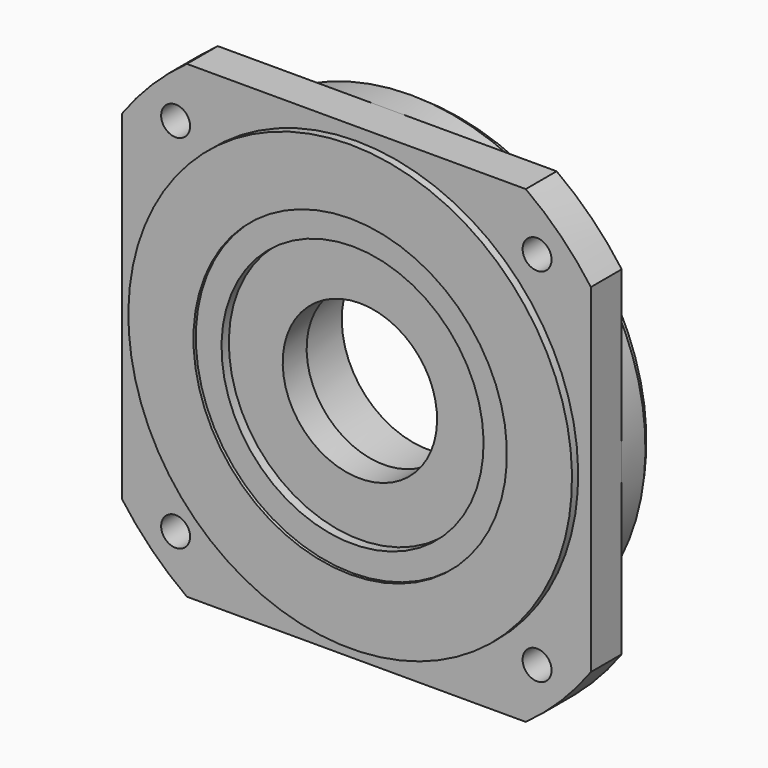
from build123d import *

# Parameters (mm, degrees)
F2_R            = 7.5
F3_DEPTH        = 25.4
F3_COPIES_COUNT = 4
F4_R            = 12.7


# Not quite as in the source:
# - a pattern or mirror of a feature is missing from the dataset's text; its kind, count and spacing are read off the source's solid


with BuildPart() as f1:
    # F0 (on Right) → F1 (revolve)
    with BuildSketch(Plane.YZ):
        Polygon((23.9776, 150), (3.9878, 150), (3.9878, 114.9985), (0, 114.9985), (0, 81.2514126301), (1.524, 81.2514126301), (1.524, 67.9329782724), (6.2865, 67.9329782724), (6.2865, 40.0177), (21.7932, 40.0177), (21.7932, 45.0088), (50.8, 45.0088), (50.8, 51.3588), (12.7, 54.6921180803), (12.7, 113.4999), (44.1452, 113.4999), (44.1452, 118.2624), (39.37, 118.2624), (39.37, 121.5898), (23.9776, 121.5898), align=None)
    revolve(axis=Axis((0, 63.4710703942, 0), (0, 1, 0)))

    # F2 (on face) → F3 (cut)
    with BuildSketch(Plane.XZ.offset(-3.9878)):
        with Locations((-93.6910121111, 93.6910121111)):
            Circle(F2_R)
        with BuildLine():
            Line((-111.0230386257, 169.054677367), (-111.0230386257, 121.5898))
            Line((-111.0230386257, 121.5898), (-87.8403127041, 121.5898))
            ThreePointArc((-87.8403127041, 121.5898), (0, 150), (87.8403127041, 121.5898))
            Line((87.8403127041, 121.5898), (147.7070748806, 121.5898))
            Line((147.7070748806, 121.5898), (147.7070748806, 169.054677367))
            Line((147.7070748806, 169.054677367), (-111.0230386257, 169.054677367))
        make_face()
        with BuildLine():
            ThreePointArc((87.8403127041, 121.5898), (0, 150), (-87.8403127041, 121.5898))
            Line((-87.8403127041, 121.5898), (87.8403127041, 121.5898))
        make_face()
    f3 = extrude(amount=-F3_DEPTH, mode=Mode.SUBTRACT)

    # F3_copies: F3 ×4 about axis
    f3_copies_axis = Axis((0, 0, 0), (0, 1, 0))
    for i in range(1, F3_COPIES_COUNT):
        add(f3.rotate(f3_copies_axis, i * 360 / F3_COPIES_COUNT), mode=Mode.SUBTRACT)

    # F4
    f4_edges = [f1.edges().sort_by_distance(p)[0] for p in [
        (0, 12.7, -113.4999),
        (0, 12.7, -54.692118),
    ]]
    fillet(f4_edges, radius=F4_R)


solid = f1.part
